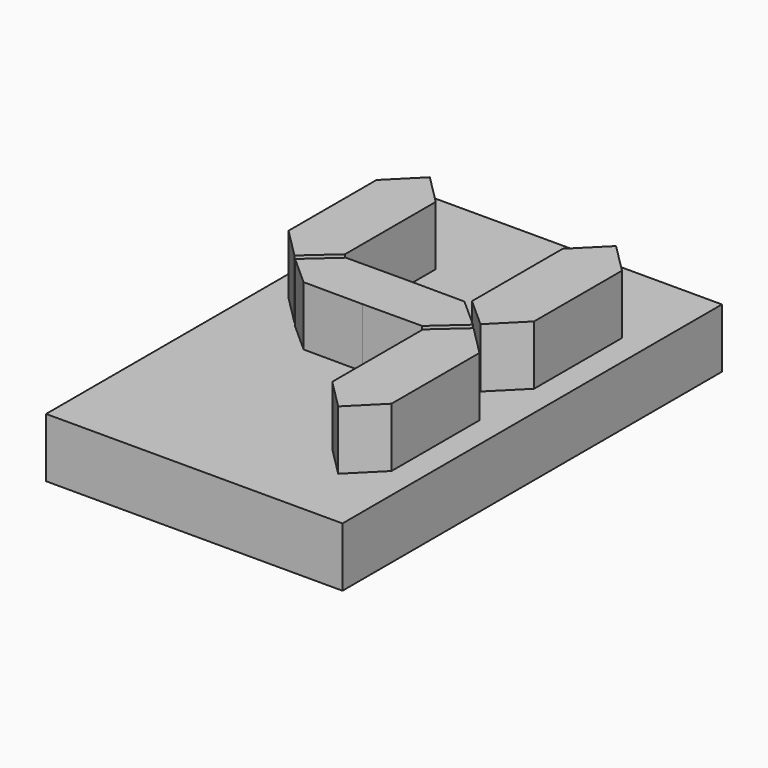
from build123d import *

# Parameters (mm, degrees)
F0_W     = 10
F0_H     = 16
F1_DEPTH = 2
F3_DEPTH = 2


# Not quite as in the source:
# - ends of sketch curves that miss each other by under 0.0002 mm in the source are joined


with BuildPart() as f1:
    # F0 (on Top) → F1 (new body)
    with BuildSketch(Plane.XY):
        Rectangle(F0_W, F0_H)
    extrude(amount=F1_DEPTH)

    # F2 (on face) → F3 (join)
    with BuildSketch(Plane.XY.offset(2)):
        Polygon((-2.1414213562, 4.8585786438), (-3.1414213562, 5.8585786438), (-4.1414213562, 4.8585786438), (-4.1414213562, 1.1507223826), (-3.1374518146, 0.1453992321), (-2.1414213562, 1.0335195075), align=None)
        Polygon((2, 0.891659756), (2.00782e-05, 0.9006214721), (-2, 0.891659756), (-3, 0), (-2, -0.891659756), (-2.00782e-05, -0.9006214721), (2, -0.891659756), (3, 0), align=None)
        Polygon((4.1414213562, 4.8585786438), (3.1414213562, 5.8585786438), (2.1414213562, 4.8585786438), (2.1414213562, 1.0335195075), (3.1374518146, 0.1453992321), (4.1414213562, 1.1507223826), align=None)
        Polygon((3.1374518146, -0.1453992321), (2.1414213562, -1.0335195075), (2.1414213562, -4.8585786438), (3.1414213562, -5.8585786438), (4.1414213562, -4.8585786438), (4.1414213562, -1.1507223826), align=None)
    extrude(amount=F3_DEPTH)


solid = f1.part
